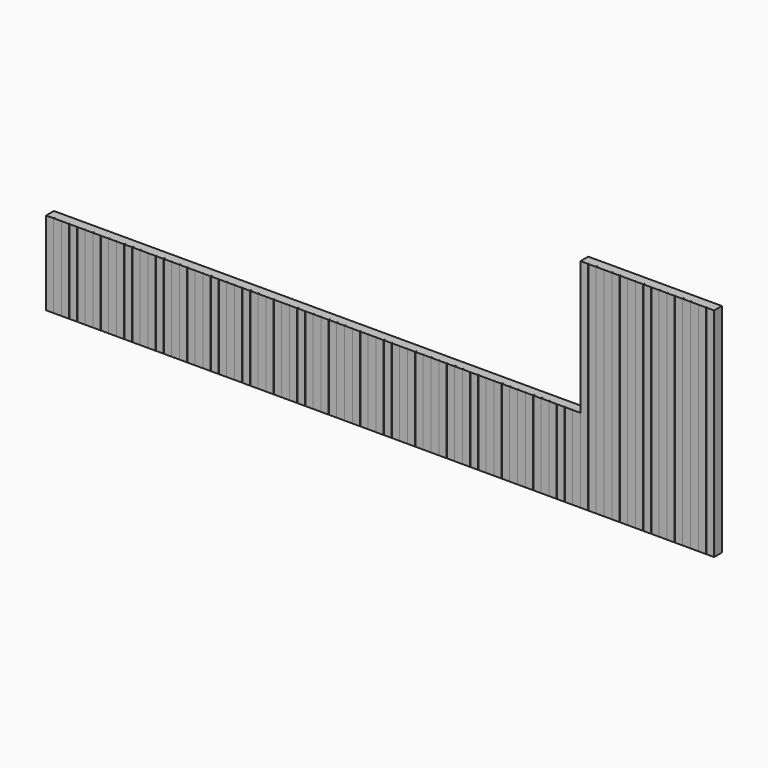
from build123d import *

# Parameters (mm, degrees)
F0_W     = 38.1
F0_H     = 38.1
F0_H_2   = 368.3
F0_H_3   = 228.6
F0_W_2   = 4838.7
F0_W_3   = 2362.2
F1_DEPTH = 152.4
F2_W     = 139.7
F2_H     = 3962.4
F2_H_2   = 1524
F2_W_2   = 134.62
F3_DEPTH = 25.4


with BuildPart() as f1:
    # F0 (on Front) → F1 (new body)
    with BuildSketch(Plane.XZ):
        Polygon((0, 1524), (0, 0), (4876.8, 0), (4876.8, 38.1), (38.1, 38.1), (38.1, 406.4), (38.1, 444.5), (38.1, 812.8), (38.1, 850.9), (38.1, 1219.2), (38.1, 1257.3), (38.1, 1485.9), (4876.8, 1485.9), (4876.8, 1524), align=None)
        with Locations((4895.85, 19.05)):
            Rectangle(F0_W, F0_H)
        with Locations((4895.85, 1504.95)):
            Rectangle(F0_W, F0_H)
        Polygon((4914.9, 38.1), (4914.9, 0), (12192, 0), (12192, 3962.4), (9753.6, 3962.4), (9753.6, 1524), (4914.9, 1524), (4914.9, 1485.9), (9753.6, 1485.9), (9791.7, 1485.9), (9791.7, 1524), (9791.7, 1892.3), (9791.7, 1930.4), (9791.7, 2298.7), (9791.7, 2336.8), (9791.7, 2705.1), (9791.7, 2743.2), (9791.7, 3111.5), (9791.7, 3149.6), (9791.7, 3517.9), (9791.7, 3556), (9791.7, 3924.3), (12153.9, 3924.3), (12153.9, 3556), (12153.9, 3517.9), (12153.9, 3149.6), (12153.9, 3111.5), (12153.9, 2743.2), (12153.9, 2705.1), (12153.9, 2336.8), (12153.9, 2298.7), (12153.9, 1930.4), (12153.9, 1892.3), (12153.9, 1524), (12153.9, 1485.9), (12153.9, 1257.3), (12153.9, 1219.2), (12153.9, 850.9), (12153.9, 812.8), (12153.9, 444.5), (12153.9, 425.45), (12153.9, 406.4), (12153.9, 38.1), (9791.7, 38.1), (9753.6, 38.1), align=None)
        with Locations((4895.85, 222.25)):
            Rectangle(F0_W, F0_H_2)
        with Locations((4895.85, 1371.6)):
            Rectangle(F0_W, F0_H_3)
        with Locations((2457.45, 425.45)):
            Rectangle(F0_W_2, F0_H)
        with Locations((4895.85, 425.45)):
            Rectangle(F0_W, F0_H)
        with Locations((4895.85, 1238.25)):
            Rectangle(F0_W, F0_H)
        with Locations((2457.45, 1238.25)):
            Rectangle(F0_W_2, F0_H)
        with Locations((9772.65, 222.25)):
            Rectangle(F0_W, F0_H_2)
        with Locations((7334.25, 425.45)):
            Rectangle(F0_W_2, F0_H)
        with Locations((4895.85, 628.65)):
            Rectangle(F0_W, F0_H_2)
        with Locations((9772.65, 1371.6)):
            Rectangle(F0_W, F0_H_3)
        with Locations((7334.25, 1238.25)):
            Rectangle(F0_W_2, F0_H)
        with Locations((4895.85, 1035.05)):
            Rectangle(F0_W, F0_H_2)
        with Locations((9772.65, 425.45)):
            Rectangle(F0_W, F0_H)
        with Locations((2457.45, 831.85)):
            Rectangle(F0_W_2, F0_H)
        with Locations((4895.85, 831.85)):
            Rectangle(F0_W, F0_H)
        with Locations((10972.8, 1504.95)):
            Rectangle(F0_W_3, F0_H)
        with Locations((9772.65, 1238.25)):
            Rectangle(F0_W, F0_H)
        Polygon((9791.7, 444.5), (9791.7, 406.4), (12153.9, 406.4), (12153.9, 425.45), (12153.9, 444.5), align=None)
        with Locations((9772.65, 628.65)):
            Rectangle(F0_W, F0_H_2)
        with Locations((7334.25, 831.85)):
            Rectangle(F0_W_2, F0_H)
        with Locations((10972.8, 1238.25)):
            Rectangle(F0_W_3, F0_H)
        with Locations((9772.65, 1035.05)):
            Rectangle(F0_W, F0_H_2)
        with Locations((9772.65, 831.85)):
            Rectangle(F0_W, F0_H)
        with Locations((10972.8, 1911.35)):
            Rectangle(F0_W_3, F0_H)
        with Locations((10972.8, 831.85)):
            Rectangle(F0_W_3, F0_H)
        with Locations((10972.8, 2317.75)):
            Rectangle(F0_W_3, F0_H)
        with Locations((10972.8, 2724.15)):
            Rectangle(F0_W_3, F0_H)
        with Locations((10972.8, 3130.55)):
            Rectangle(F0_W_3, F0_H)
        with Locations((10972.8, 3536.95)):
            Rectangle(F0_W_3, F0_H)
    extrude(amount=F1_DEPTH)

    # F2 (on face) → F3 (join)
    with BuildSketch(Plane.XZ.offset(152.4)):
        with Locations((9823.45, 1981.2)):
            Rectangle(F2_W, F2_H)
        with Locations((9966.96, 1981.2)):
            Rectangle(F2_W, F2_H)
        with Locations((10110.47, 1981.2)):
            Rectangle(F2_W, F2_H)
        with Locations((10253.98, 1981.2)):
            Rectangle(F2_W, F2_H)
        with Locations((10397.49, 1981.2)):
            Rectangle(F2_W, F2_H)
        with Locations((10541, 1981.2)):
            Rectangle(F2_W, F2_H)
        with Locations((10684.51, 1981.2)):
            Rectangle(F2_W, F2_H)
        with Locations((10828.02, 1981.2)):
            Rectangle(F2_W, F2_H)
        with Locations((10971.53, 1981.2)):
            Rectangle(F2_W, F2_H)
        with Locations((11115.04, 1981.2)):
            Rectangle(F2_W, F2_H)
        with Locations((11258.55, 1981.2)):
            Rectangle(F2_W, F2_H)
        with Locations((11402.06, 1981.2)):
            Rectangle(F2_W, F2_H)
        with Locations((11545.57, 1981.2)):
            Rectangle(F2_W, F2_H)
        with Locations((11689.08, 1981.2)):
            Rectangle(F2_W, F2_H)
        with Locations((11832.59, 1981.2)):
            Rectangle(F2_W, F2_H)
        with Locations((11976.1, 1981.2)):
            Rectangle(F2_W, F2_H)
        with Locations((12119.61, 1981.2)):
            Rectangle(F2_W, F2_H)
        with Locations((9679.94, 762)):
            Rectangle(F2_W, F2_H_2)
        with Locations((9536.43, 762)):
            Rectangle(F2_W, F2_H_2)
        with Locations((9392.92, 762)):
            Rectangle(F2_W, F2_H_2)
        with Locations((9249.41, 762)):
            Rectangle(F2_W, F2_H_2)
        with Locations((9105.9, 762)):
            Rectangle(F2_W, F2_H_2)
        with Locations((8962.39, 762)):
            Rectangle(F2_W, F2_H_2)
        with Locations((8818.88, 762)):
            Rectangle(F2_W, F2_H_2)
        with Locations((8675.37, 762)):
            Rectangle(F2_W, F2_H_2)
        with Locations((8531.86, 762)):
            Rectangle(F2_W, F2_H_2)
        with Locations((8388.35, 762)):
            Rectangle(F2_W, F2_H_2)
        with Locations((8244.84, 762)):
            Rectangle(F2_W, F2_H_2)
        with Locations((8101.33, 762)):
            Rectangle(F2_W, F2_H_2)
        with Locations((7957.82, 762)):
            Rectangle(F2_W, F2_H_2)
        with Locations((7814.31, 762)):
            Rectangle(F2_W, F2_H_2)
        with Locations((7670.8, 762)):
            Rectangle(F2_W, F2_H_2)
        with Locations((7527.29, 762)):
            Rectangle(F2_W, F2_H_2)
        with Locations((7383.78, 762)):
            Rectangle(F2_W, F2_H_2)
        with Locations((7240.27, 762)):
            Rectangle(F2_W, F2_H_2)
        with Locations((7096.76, 762)):
            Rectangle(F2_W, F2_H_2)
        with Locations((6953.25, 762)):
            Rectangle(F2_W, F2_H_2)
        with Locations((6809.74, 762)):
            Rectangle(F2_W, F2_H_2)
        with Locations((6666.23, 762)):
            Rectangle(F2_W, F2_H_2)
        with Locations((6522.72, 762)):
            Rectangle(F2_W, F2_H_2)
        with Locations((6379.21, 762)):
            Rectangle(F2_W, F2_H_2)
        with Locations((6235.7, 762)):
            Rectangle(F2_W, F2_H_2)
        with Locations((6092.19, 762)):
            Rectangle(F2_W, F2_H_2)
        with Locations((5948.68, 762)):
            Rectangle(F2_W, F2_H_2)
        with Locations((5805.17, 762)):
            Rectangle(F2_W, F2_H_2)
        with Locations((5661.66, 762)):
            Rectangle(F2_W, F2_H_2)
        with Locations((5518.15, 762)):
            Rectangle(F2_W, F2_H_2)
        with Locations((5374.64, 762)):
            Rectangle(F2_W, F2_H_2)
        with Locations((5231.13, 762)):
            Rectangle(F2_W, F2_H_2)
        with Locations((5087.62, 762)):
            Rectangle(F2_W, F2_H_2)
        with Locations((4944.11, 762)):
            Rectangle(F2_W, F2_H_2)
        with Locations((4800.6, 762)):
            Rectangle(F2_W, F2_H_2)
        with Locations((4657.09, 762)):
            Rectangle(F2_W, F2_H_2)
        with Locations((4513.58, 762)):
            Rectangle(F2_W, F2_H_2)
        with Locations((4370.07, 762)):
            Rectangle(F2_W, F2_H_2)
        with Locations((4226.56, 762)):
            Rectangle(F2_W, F2_H_2)
        with Locations((4083.05, 762)):
            Rectangle(F2_W, F2_H_2)
        with Locations((3939.54, 762)):
            Rectangle(F2_W, F2_H_2)
        with Locations((3796.03, 762)):
            Rectangle(F2_W, F2_H_2)
        with Locations((3652.52, 762)):
            Rectangle(F2_W, F2_H_2)
        with Locations((3509.01, 762)):
            Rectangle(F2_W, F2_H_2)
        with Locations((3365.5, 762)):
            Rectangle(F2_W, F2_H_2)
        with Locations((3221.99, 762)):
            Rectangle(F2_W, F2_H_2)
        with Locations((3078.48, 762)):
            Rectangle(F2_W, F2_H_2)
        with Locations((2934.97, 762)):
            Rectangle(F2_W, F2_H_2)
        with Locations((2791.46, 762)):
            Rectangle(F2_W, F2_H_2)
        with Locations((2647.95, 762)):
            Rectangle(F2_W, F2_H_2)
        with Locations((2504.44, 762)):
            Rectangle(F2_W, F2_H_2)
        with Locations((2360.93, 762)):
            Rectangle(F2_W, F2_H_2)
        with Locations((2217.42, 762)):
            Rectangle(F2_W, F2_H_2)
        with Locations((2073.91, 762)):
            Rectangle(F2_W, F2_H_2)
        with Locations((1930.4, 762)):
            Rectangle(F2_W, F2_H_2)
        with Locations((1786.89, 762)):
            Rectangle(F2_W, F2_H_2)
        with Locations((1643.38, 762)):
            Rectangle(F2_W, F2_H_2)
        with Locations((1499.87, 762)):
            Rectangle(F2_W, F2_H_2)
        with Locations((1356.36, 762)):
            Rectangle(F2_W, F2_H_2)
        with Locations((1212.85, 762)):
            Rectangle(F2_W, F2_H_2)
        with Locations((1069.34, 762)):
            Rectangle(F2_W, F2_H_2)
        with Locations((925.83, 762)):
            Rectangle(F2_W, F2_H_2)
        with Locations((782.32, 762)):
            Rectangle(F2_W, F2_H_2)
        with Locations((638.81, 762)):
            Rectangle(F2_W, F2_H_2)
        with Locations((495.3, 762)):
            Rectangle(F2_W, F2_H_2)
        with Locations((351.79, 762)):
            Rectangle(F2_W, F2_H_2)
        with Locations((208.28, 762)):
            Rectangle(F2_W, F2_H_2)
        with Locations((67.31, 762)):
            Rectangle(F2_W_2, F2_H_2)
    extrude(amount=F3_DEPTH)


solid = f1.part
